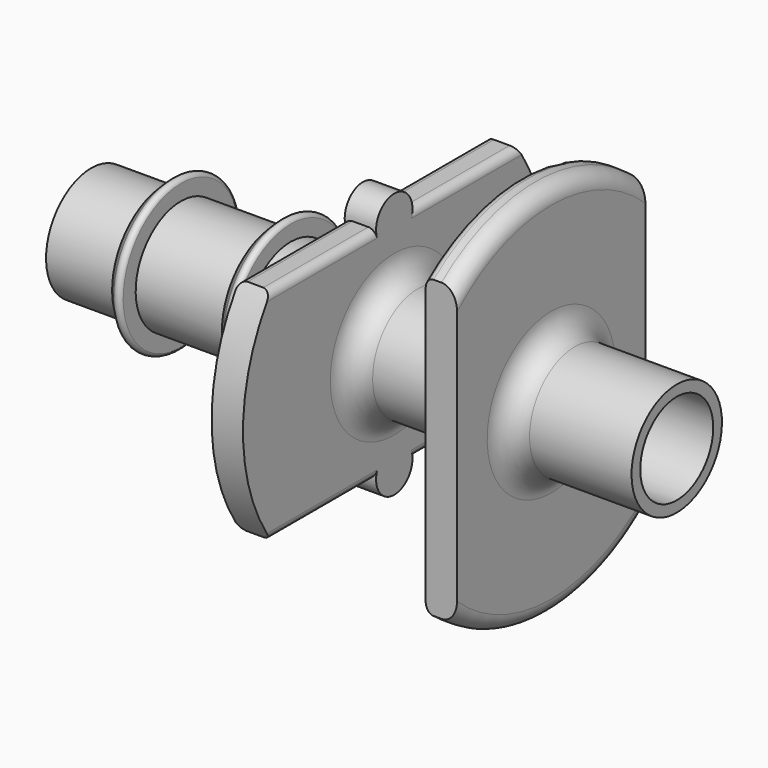
from build123d import *

# Parameters (mm, degrees)
F2_R     = 1.5
F3_SIZE2 = 0.2886751346
F3_SIZE  = 0.5
F5_DEPTH = 3.9
F7_DEPTH = 5
F8_R     = 0.5
F9_R     = 1
F10_R    = 0.5


with BuildPart() as f1:
    # F0 (on Front) → F1 (revolve)
    with BuildSketch(Plane.XZ):
        with BuildLine():
            Line((6, 3.6), (1, 3.6))
            Line((1, 3.6), (1, 2.25))
            Line((1, 2.25), (38.6, 2.9063104413))
            Line((38.6, 2.9063104413), (38.6, 3.6))
            Line((38.6, 3.6), (30.6, 3.6))
            Line((30.6, 3.6), (30.6, 12.05))
            Line((30.6, 12.05), (28.6, 12.05))
            Line((28.6, 12.05), (28.6, 3.6))
            Line((28.6, 3.6), (20.6, 3.6))
            Line((20.6, 3.6), (20.6, 12.05))
            Line((20.6, 12.05), (18.6, 12.05))
            Line((18.6, 12.05), (18.6, 3.6))
            Line((18.6, 3.6), (14, 3.6))
            Line((14, 3.6), (14, 4.6))
            ThreePointArc((14, 4.6), (13.7863585166, 4.8062210018), (13.5, 4.7276806616))
            Line((13.5, 4.7276806616), (13, 4.2276806616))
            Line((13, 4.2276806616), (13, 3.6))
            Line((13, 3.6), (7, 3.6))
            Line((7, 3.6), (7, 4.6))
            ThreePointArc((7, 4.6), (6.7863585166, 4.8062210018), (6.5, 4.7276806616))
            Line((6.5, 4.7276806616), (6, 4.2276806616))
            Line((6, 4.2276806616), (6, 3.6))
        make_face()
    revolve(axis=Axis((21.4299485087, 0, 0), (1, 0, 0)))

    # F2
    f2_edges = [f1.edges().sort_by_distance(p)[0] for p in [
        (18.6, 0, -3.6),
        (20.6, 0, -3.6),
        (28.6, 0, -3.6),
        (30.6, 0, -3.6),
    ]]
    fillet(f2_edges, radius=F2_R)

    # F3
    f3_edges = [f1.edges().sort_by_distance(p)[0] for p in [
        (1, 0, -3.6),
    ]]
    chamfer(f3_edges, length=F3_SIZE, length2=F3_SIZE2)

    # F4 (on face) → F5 (cut)
    with BuildSketch(Plane.YZ.offset(30.6)):
        with BuildLine():
            ThreePointArc((12.05, 0), (10.853052566, 5.2358141678), (7.5, 9.4314633011))
            Line((7.5, 9.4314633011), (7.5, -9.4314633011))
            ThreePointArc((7.5, -9.4314633011), (10.853052566, -5.2358141678), (12.05, 0))
        make_face()
        with BuildLine():
            Line((-7.5, -9.4314633011), (-7.5, 9.4314633011))
            ThreePointArc((-7.5, 9.4314633011), (-12.05, 0), (-7.5, -9.4314633011))
        make_face()
    extrude(amount=-F5_DEPTH, mode=Mode.SUBTRACT)

    # F6 (on face) → F7 (cut)
    with BuildSketch(Plane.YZ.offset(20.6)):
        with BuildLine():
            Line((-9.8082873123, 7), (-1.45, 7))
            ThreePointArc((-1.45, 7), (0, 8.45), (1.45, 7))
            Line((1.45, 7), (9.8082873123, 7))
            ThreePointArc((9.8082873123, 7), (0, 12.05), (-9.8082873123, 7))
        make_face()
        with BuildLine():
            Line((-1.45, -7), (-9.8082873123, -7))
            ThreePointArc((-9.8082873123, -7), (0, -12.05), (9.8082873123, -7))
            Line((9.8082873123, -7), (1.45, -7))
            ThreePointArc((1.45, -7), (0, -8.45), (-1.45, -7))
        make_face()
    extrude(amount=-F7_DEPTH, mode=Mode.SUBTRACT)

    # F8
    f8_edges = [f1.edges().sort_by_distance(p)[0] for p in [
        (28.6, 0, -12.05),
        (28.6, 0, 12.05),
    ]]
    fillet(f8_edges, radius=F8_R)

    # F9
    f9_edges = [f1.edges().sort_by_distance(p)[0] for p in [
        (30.6, 0, 12.05),
        (30.6, 0, -12.05),
    ]]
    fillet(f9_edges, radius=F9_R)

    # F10
    f10_edges = [f1.edges().sort_by_distance(p)[0] for p in [
        (18.6, 5.629144, 7),
        (20.6, 5.629144, 7),
        (20.6, -5.629144, 7),
        (18.6, -5.629144, 7),
        (18.6, 5.629144, -7),
        (20.6, 5.629144, -7),
        (18.6, -5.629144, -7),
        (20.6, -5.629144, -7),
    ]]
    fillet(f10_edges, radius=F10_R)


solid = f1.part
